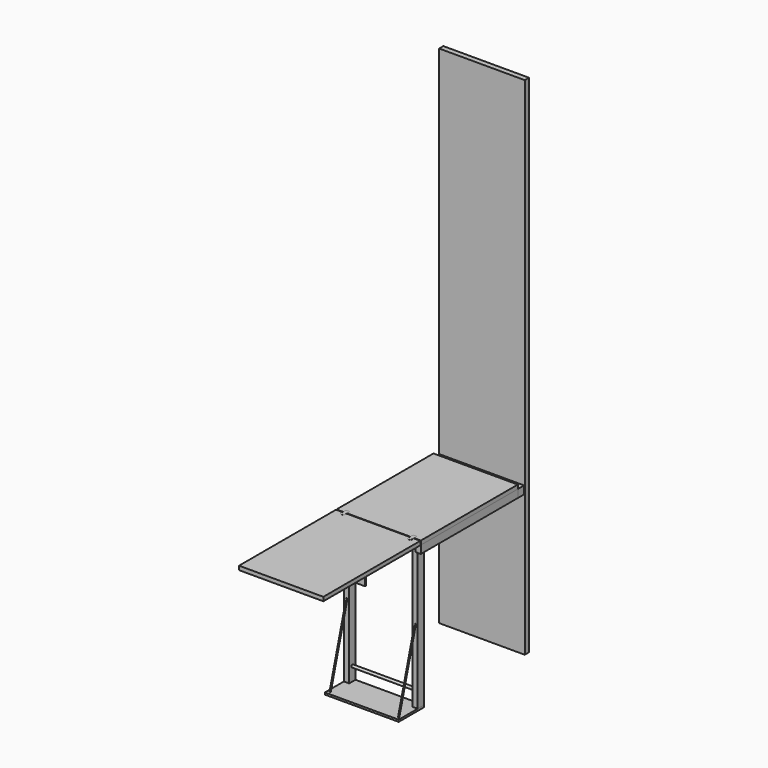
from build123d import *

# Parameters (mm, degrees)
F0_W           = 412.75
F0_H           = 2438.4
F1_DEPTH       = 25.4
F3_W           = 406.4
F3_H           = 38.1
F4_DEPTH       = 38.1
F5_W           = 406.4
F5_H           = 18.25625
F6_DEPTH       = 577.85
F7_W           = 25.4
F7_H           = 38.1
F8_DEPTH       = 584.2
F10_DEPTH      = 330.2
F10_DEPTH_BACK = 254
F11_W          = 304.8
F11_H          = 38.1
F12_DEPTH      = 6.35
F14_DEPTH      = 508
F15_W          = 329.3162656754
F15_H          = 914.4
F16_DEPTH      = 9.525
F17_W          = 304.8
F17_H          = 584.2
F18_DEPTH      = 9.525
F20_DEPTH      = 25.4
F21_W          = 406.4
F21_H          = 584.2
F22_DEPTH      = 19.05
F23_W          = 25.4
F23_H          = 38.1
F24_DEPTH      = 717.55
F25_W          = 355.6
F25_H          = 152.4
F26_DEPTH      = 9.525
F27_W          = 25.4
F27_H          = 25.4
F28_DEPTH      = 38.1
F34_R          = 2.54
F36_R          = 6.35
F37_DEPTH      = 304.8
F39_W          = 50.8
F39_H          = 38.1
F40_DEPTH      = 6.35
F42_DEPTH      = 0.254


with BuildPart() as f1:
    # F0 (on Front) → F1 (new body)
    with BuildSketch(Plane.XZ):
        with Locations((206.375, 1219.2)):
            Rectangle(F0_W, F0_H)
    extrude(amount=F1_DEPTH)


with BuildPart() as f4:
    # F3 (on face) → F4 (new body)
    with BuildSketch(Plane.XZ.offset(25.4)):
        with Locations((206.375, 698.5)):
            Rectangle(F3_W, F3_H)
    extrude(amount=F4_DEPTH)

    # F27 (on face) → F28 (cut, through all)
    with BuildSketch(Plane(origin=(0, 0, 679.45), x_dir=(1, 0, 0), z_dir=(0, 0, -1))):
        with Locations((41.275, 50.8)):
            Rectangle(F27_W, F27_H)
        with Locations((371.475, 50.8)):
            Rectangle(F27_W, F27_H)
    extrude(amount=-F28_DEPTH, mode=Mode.SUBTRACT)


with BuildPart() as f6:
    # F5 (on face) → F6 (new body, through all)
    with BuildSketch(Plane.XY.offset(717.55)):
        with Locations((206.375, -34.528125)):
            Rectangle(F5_W, F5_H)
    extrude(amount=F6_DEPTH)


with BuildPart() as f6b:
    # F5 (on face) → F6, piece 2 (new body, through all)
    with BuildSketch(Plane.XY.offset(717.55)):
        with Locations((206.375, -54.371875)):
            Rectangle(F5_W, F5_H)
    extrude(amount=F6_DEPTH)


with BuildPart() as f8:
    # F7 (on face) → F8 (new body)
    with BuildSketch(Plane.XZ.offset(63.5)):
        with Locations((15.875, 698.5)):
            Rectangle(F7_W, F7_H)
    extrude(amount=F8_DEPTH)


with BuildPart() as f8b:
    # F7 (on face) → F8, piece 2 (new body)
    with BuildSketch(Plane.XZ.offset(63.5)):
        with Locations((396.875, 698.5)):
            Rectangle(F7_W, F7_H)
    extrude(amount=F8_DEPTH)


with BuildPart() as f10:
    # F9 (on face) → F10 (new body, two sides)
    with BuildSketch(Plane.XZ.offset(647.7)) as f10_sk:
        Polygon((79.375, 717.55), (53.975, 717.55), (53.975, 679.45), (79.375, 679.45), (79.375, 692.15), (73.025, 692.15), (73.025, 704.85), (79.375, 704.85), align=None)
    extrude(amount=F10_DEPTH)
    extrude(f10_sk.sketch, amount=-F10_DEPTH_BACK)


with BuildPart() as f10b:
    # F9 (on face) → F10, piece 2 (new body, two sides)
    with BuildSketch(Plane.XZ.offset(647.7)) as f10_2_sk:
        Polygon((358.775, 717.55), (333.375, 717.55), (333.375, 704.85), (339.725, 704.85), (339.725, 692.15), (333.375, 692.15), (333.375, 679.45), (358.775, 679.45), align=None)
    extrude(amount=F10_DEPTH)
    extrude(f10_2_sk.sketch, amount=-F10_DEPTH_BACK)


with BuildPart() as f12:
    # F11 (on face) → F12 (new body)
    with BuildSketch(Plane.XZ.offset(977.9)):
        with Locations((206.375, 698.5)):
            Rectangle(F11_W, F11_H)
    extrude(amount=F12_DEPTH)

    # F19 (on face) → F20 (cut)
    with BuildSketch(Plane.XZ.offset(984.25)):
        with BuildLine():
            Line((273.05, 698.5), (139.7, 698.5))
            ThreePointArc((139.7, 698.5), (132.9648079092, 695.7101920908), (130.175, 688.975))
            Line((130.175, 688.975), (130.175, 685.8))
            ThreePointArc((130.175, 685.8), (128.3151280605, 681.3098719395), (123.825, 679.45))
            Line((123.825, 679.45), (104.5370513368, 679.45))
            Line((104.5370513368, 679.45), (95.1471963692, 663.4348630905))
            Line((95.1471963692, 663.4348630905), (306.0875535011, 663.4348630905))
            Line((306.0875535011, 663.4348630905), (306.0875535011, 679.45))
            Line((306.0875535011, 679.45), (288.925, 679.45))
            ThreePointArc((288.925, 679.45), (284.4348719395, 681.3098719395), (282.575, 685.8))
            Line((282.575, 685.8), (282.575, 688.975))
            ThreePointArc((282.575, 688.975), (279.7851920908, 695.7101920908), (273.05, 698.5))
        make_face()
    extrude(amount=-F20_DEPTH, mode=Mode.SUBTRACT)

    # F39 (on face) → F40 (join)
    with BuildSketch(Plane.XZ.offset(984.25)):
        with Locations((384.175, 698.5)):
            Rectangle(F39_W, F39_H)
        with Locations((28.575, 698.5)):
            Rectangle(F39_W, F39_H)
    extrude(amount=-F40_DEPTH)


with BuildPart() as f14:
    # F13 (on face) → F14 (new body)
    with BuildSketch(Plane.XZ.offset(647.7)):
        Polygon((98.425, 717.55), (79.375, 717.55), (79.375, 704.85), (73.025, 704.85), (73.025, 692.15), (79.375, 692.15), (79.375, 679.45), (98.425, 679.45), align=None)
    extrude(amount=-F14_DEPTH)


with BuildPart() as f14b:
    # F13 (on face) → F14, piece 2 (new body)
    with BuildSketch(Plane.XZ.offset(647.7)):
        Polygon((333.375, 704.85), (333.375, 717.55), (314.325, 717.55), (314.325, 679.45), (333.375, 679.45), (333.375, 692.15), (339.725, 692.15), (339.725, 704.85), align=None)
    extrude(amount=-F14_DEPTH)


with BuildPart() as f16_tool:
    # F15 (on face) → F16 (new body)
    with BuildSketch(Plane(origin=(0, 0, 679.45), x_dir=(1, 0, 0), z_dir=(0, 0, -1))):
        with Locations((208.811474897, 520.7)):
            Rectangle(F15_W, F15_H)
    extrude(amount=-F16_DEPTH)


with BuildPart() as f10_1:
    add(f10.part)

    # F16: cut by f16_tool
    add(f16_tool.part, mode=Mode.SUBTRACT)


with BuildPart() as f10b_1:
    add(f10b.part)

    # F16: cut by f16_tool
    add(f16_tool.part, mode=Mode.SUBTRACT)


with BuildPart() as f14_1:
    add(f14.part)

    # F16: cut by f16_tool
    add(f16_tool.part, mode=Mode.SUBTRACT)


with BuildPart() as f14b_1:
    add(f14b.part)

    # F16: cut by f16_tool
    add(f16_tool.part, mode=Mode.SUBTRACT)


with BuildPart() as f18:
    # F17 (on face) → F18 (new body, through all)
    with BuildSketch(Plane(origin=(0, 0, 679.45), x_dir=(1, 0, 0), z_dir=(0, 0, -1))):
        with Locations((206.375, 355.6)):
            Rectangle(F17_W, F17_H)
    extrude(amount=-F18_DEPTH)


with BuildPart() as f22:
    # F21 (on face) → F22 (new body)
    with BuildSketch(Plane.XY.offset(717.55)):
        with Locations((206.375, -355.6)):
            Rectangle(F21_W, F21_H)
    extrude(amount=F22_DEPTH)


with BuildPart() as f22b:
    # F21 (on face) → F22, piece 2 (new body)
    with BuildSketch(Plane.XY.offset(717.55)):
        with Locations((206.375, -942.975)):
            Rectangle(F21_W, F21_H)
    extrude(amount=F22_DEPTH)


with BuildPart() as f24:
    # F23 (on face) → F24 (new body, through all)
    with BuildSketch(Plane(origin=(0, 0, 717.55), x_dir=(1, 0, 0), z_dir=(0, 0, -1))):
        with Locations((41.275, 615.95)):
            Rectangle(F23_W, F23_H)
    extrude(amount=F24_DEPTH)


with BuildPart() as f24b:
    # F23 (on face) → F24, piece 2 (new body, through all)
    with BuildSketch(Plane(origin=(0, 0, 717.55), x_dir=(1, 0, 0), z_dir=(0, 0, -1))):
        with Locations((371.475, 615.95)):
            Rectangle(F23_W, F23_H)
    extrude(amount=F24_DEPTH)


with BuildPart() as f26:
    # F25 (on face) → F26 (new body)
    with BuildSketch(Plane(origin=(0, 0, 0), x_dir=(1, 0, 0), z_dir=(0, 0, -1))):
        with Locations((206.375, 673.1)):
            Rectangle(F25_W, F25_H)
    extrude(amount=-F26_DEPTH)


with BuildPart() as f35:
    # F35: sweep along a path in F32
    with BuildLine(Plane.YZ.offset(41.275)) as f35_path:
        Line((-733.3971261978, 9.525), (-635.2745294571, 358.1574260011))
        Line((-635.2745294571, 358.1574260011), (-623.6042869703, 399.622135307))
    # F34 (on face) → F35 (sweep)
    with BuildSketch(Plane.XY.offset(9.525)):
        with Locations((41.275, -733.3971261978)):
            Circle(F34_R)
        with Locations((371.475, -733.3971261978)):
            Circle(F34_R)
    sweep(path=f35_path.line)


with BuildPart() as f37:
    # F36 (on face) → F37 (new body, through all)
    with BuildSketch(Plane.YZ.offset(53.975)):
        with Locations((-615.95, 76.2)):
            Circle(F36_R)
    extrude(amount=F37_DEPTH)


with BuildPart() as f42:
    # F41 (on face) → F42 (new body)
    with BuildSketch(Plane.XY.offset(736.6)):
        with BuildLine():
            Line((47.625, -630.2375), (41.275, -630.2375))
            ThreePointArc((41.275, -630.2375), (36.7848719395, -632.0973719395), (34.925, -636.5875))
            Line((34.925, -636.5875), (34.925, -661.9875))
            ThreePointArc((34.925, -661.9875), (36.7848719395, -666.4776280605), (41.275, -668.3375))
            Line((41.275, -668.3375), (47.625, -668.3375))
            ThreePointArc((47.625, -668.3375), (52.1151280605, -666.4776280605), (53.975, -661.9875))
            Line((53.975, -661.9875), (53.975, -636.5875))
            ThreePointArc((53.975, -636.5875), (52.1151280605, -632.0973719395), (47.625, -630.2375))
        make_face()
    extrude(amount=F42_DEPTH)


with BuildPart() as f42b:
    # F41 (on face) → F42, piece 2 (new body)
    with BuildSketch(Plane.XY.offset(736.6)):
        with BuildLine():
            Line((371.475, -630.2375), (365.125, -630.2375))
            ThreePointArc((365.125, -630.2375), (360.6348719395, -632.0973719395), (358.775, -636.5875))
            Line((358.775, -636.5875), (358.775, -663.5982181152))
            ThreePointArc((358.775, -663.5982181152), (360.6348719395, -668.0883461758), (365.125, -669.9482181152))
            Line((365.125, -669.9482181152), (371.475, -669.9482181152))
            ThreePointArc((371.475, -669.9482181152), (375.9651280605, -668.0883461758), (377.825, -663.5982181152))
            Line((377.825, -663.5982181152), (377.825, -636.5875))
            ThreePointArc((377.825, -636.5875), (375.9651280605, -632.0973719395), (371.475, -630.2375))
        make_face()
    extrude(amount=F42_DEPTH)


solid = Compound([f1.part, f4.part, f8.part, f8b.part, f12.part, f10_1.part, f10b_1.part, f14_1.part, f14b_1.part, f18.part, f22.part, f22b.part, f24.part, f24b.part, f26.part, f35.part, f37.part, f42.part, f42b.part])
